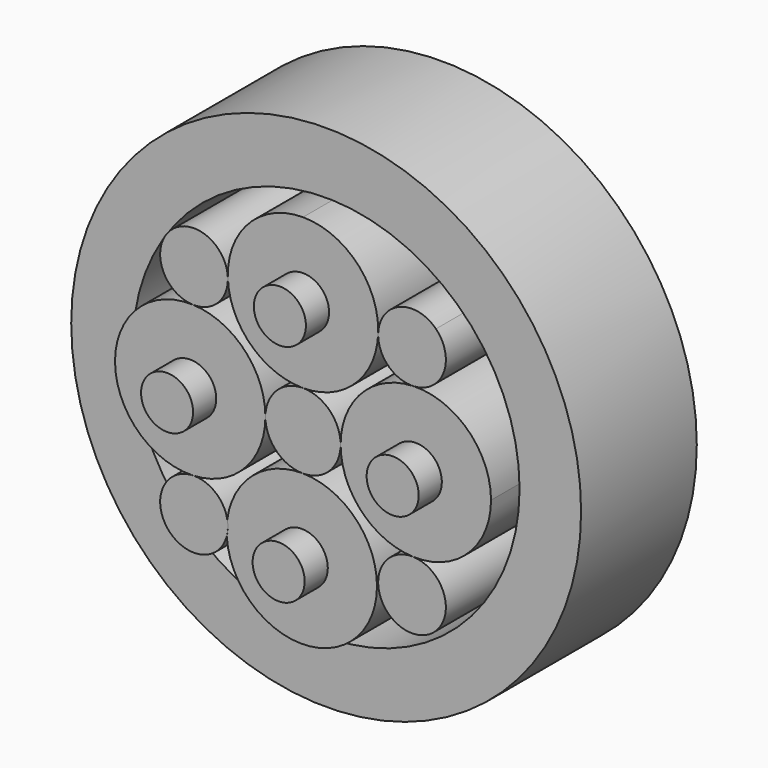
from build123d import *

# Parameters (mm, degrees)
F0_R      = 4.5
F1_DEPTH  = 35
F2_DEPTH  = 30
F3_DEPTH  = 30
F4_DEPTH  = 35
F5_DEPTH  = 30
F6_DEPTH  = 30
F7_DEPTH  = 35
F9_DEPTH  = 35
F10_R     = 44.074281088
F10_R_2   = 33.4370635173
F11_DEPTH = 25
F12_DEPTH = 30
F13_COUNT = 4
F14_DEPTH = 30


# Not quite as in the source:
# - a feature of the source that left no trace in its solid (it failed there, or was rolled back) is left out
# - a feature names something its author has since deleted; it is built from what else it names


with BuildPart() as f1:
    # F0 (on Front) → F1 (new body)
    with BuildSketch(Plane.XZ):
        with Locations((0, 19.5)):
            Circle(F0_R)
    extrude(amount=F1_DEPTH)


with BuildPart() as f2:
    # F0 (on Front) → F2 (new body)
    with BuildSketch(Plane.XZ):
        with BuildLine():
            ThreePointArc((-12.9920791749, 19.0462614041), (-9.030542571, 10.148566908), (0, 6.5))
            ThreePointArc((0, 6.5), (9.030542571, 10.148566908), (12.9920791749, 19.0462614041))
            ThreePointArc((12.9920791749, 19.0462614041), (12.9980196429, 19.2730961366), (13, 19.5))
            ThreePointArc((13, 19.5), (9.1923881501, 28.6923881607), (-1.5e-08, 32.5))
            ThreePointArc((-1.5e-08, 32.5), (-9.3514330972, 28.5305425656), (-12.9920791749, 19.0462614041))
        make_face()
        with Locations((0, 19.5)):
            Circle(F0_R, mode=Mode.SUBTRACT)
    extrude(amount=F2_DEPTH)


with BuildPart() as f3:
    # F0 (on Front) → F3 (new body)
    with BuildSketch(Plane.XZ):
        with BuildLine():
            ThreePointArc((-19.0462616463, -12.9920791833), (-10.1485669922, -9.0305426582), (-6.5, 0))
            ThreePointArc((-6.5, 0), (-10.1485669922, 9.0305426582), (-19.0462616463, 12.9920791833))
            ThreePointArc((-19.0462616463, 12.9920791833), (-28.5305425766, 9.3514330866), (-32.5, 2.269e-07))
            ThreePointArc((-32.5, 2.269e-07), (-28.5305427398, -9.351432929), (-19.0462616463, -12.9920791833))
        make_face()
        with Locations((-19.5, 0)):
            Circle(F0_R, mode=Mode.SUBTRACT)
    extrude(amount=F3_DEPTH)


with BuildPart() as f4:
    # F0 (on Front) → F4 (new body)
    with BuildSketch(Plane.XZ):
        with Locations((-19.5, 0)):
            Circle(F0_R)
    extrude(amount=F4_DEPTH)


with BuildPart() as f5:
    # F0 (on Front) → F5 (new body)
    with BuildSketch(Plane.XZ):
        with BuildLine():
            ThreePointArc((19.0462612866, 12.9920791708), (10.1485668672, 9.0305425287), (6.5, 0))
            ThreePointArc((6.5, 0), (10.1485669557, -9.0305426203), (19.0462615412, -12.9920791797))
            ThreePointArc((19.0462615412, -12.9920791797), (28.5305426203, -9.3514330443), (32.5, 0))
            ThreePointArc((32.5, 0), (28.5305425287, 9.3514331328), (19.0462612866, 12.9920791708))
        make_face()
        with Locations((19.5, 0)):
            Circle(F0_R, mode=Mode.SUBTRACT)
    extrude(amount=F5_DEPTH)


with BuildPart() as f6:
    # F0 (on Front) → F6 (new body)
    with BuildSketch(Plane.XZ):
        with BuildLine():
            ThreePointArc((12.7868825893, -19.4988353747), (9.0293664927, -10.3568174741), (-0.0710391484, -6.4996117914))
            ThreePointArc((-0.0710391484, -6.4996117914), (-8.706943876, -9.6573460577), (-13.0934155612, -17.7387445948))
            ThreePointArc((-13.0934155612, -17.7387445948), (-13.0147974373, -18.2878635968), (-12.9885127088, -18.8419588962))
            ThreePointArc((-12.9885127088, -18.8419588962), (-13.0379426477, -19.6010555008), (-13.1853976333, -20.34733159))
            ThreePointArc((-13.1853976333, -20.34733159), (-9.1521689219, -28.9377631782), (-0.355195428, -32.4980589606))
            ThreePointArc((-0.355195428, -32.4980589606), (8.928900577, -28.7413191919), (12.7868825893, -19.4988353747))
        make_face()
        with Locations((-0.2131174107, -19.4988353747)):
            Circle(F0_R, mode=Mode.SUBTRACT)
    extrude(amount=F6_DEPTH)


with BuildPart() as f7:
    # F0 (on Front) → F7 (new body)
    with BuildSketch(Plane.XZ):
        with Locations((19.5, 0)):
            Circle(F0_R)
    extrude(amount=F7_DEPTH)


with BuildPart() as f9:
    # F0 (on Front) → F9 (new body)
    with BuildSketch(Plane.XZ):
        with Locations((-0.2131174107, -19.4988353747)):
            Circle(F0_R)
    extrude(amount=F9_DEPTH)


with BuildPart() as f11:
    # F10 (on Front) → F11 (new body)
    with BuildSketch(Plane.XZ):
        Circle(F10_R)
        Circle(F10_R_2, mode=Mode.SUBTRACT)
    extrude(amount=F11_DEPTH)


with BuildPart() as f12:
    # F0 (on Front) → F12 (new body)
    with BuildSketch(Plane.XZ):
        with BuildLine():
            ThreePointArc((-12.9885127088, 18.8419588962), (-12.9894043933, 18.9441257137), (-12.9920791749, 19.0462614041))
            ThreePointArc((-12.9920791749, 19.0462614041), (-16.6966730995, 24.2881117694), (-22.9809704144, 22.9809703627))
            ThreePointArc((-22.9809704144, 22.9809703627), (-24.2881118005, 16.6966731783), (-19.0462616463, 12.9920791833))
            ThreePointArc((-19.0462616463, 12.9920791833), (-14.7758208566, 14.6313349862), (-12.9885127088, 18.8419588962))
        make_face()
    extrude(amount=F12_DEPTH)


with BuildPart() as f13_1:
    # F13: instance of F12
    add(f12.part.rotate(Axis((0, 0, 0), (0, -1, 0)), 1 * 360 / F13_COUNT))


with BuildPart() as f13_2:
    # F13: instance of F12
    add(f12.part.rotate(Axis((0, 0, 0), (0, -1, 0)), 2 * 360 / F13_COUNT))


with BuildPart() as f13_3:
    # F13: instance of F12
    add(f12.part.rotate(Axis((0, 0, 0), (0, -1, 0)), 3 * 360 / F13_COUNT))


with BuildPart() as f14:
    # F0 (on Front) → F14 (new body)
    with BuildSketch(Plane.XZ):
        with BuildLine():
            ThreePointArc((-0.0710391484, -6.4996117914), (4.5710089442, -4.6212419578), (6.5, 0))
            ThreePointArc((6.5, 0), (4.5961940777, 4.5961940777), (0, 6.5))
            ThreePointArc((0, 6.5), (-4.5961940777, 4.5961940777), (-6.5, 0))
            ThreePointArc((-6.5, 0), (-4.6212419578, -4.5710089442), (-0.0710391484, -6.4996117914))
        make_face()
    extrude(amount=F14_DEPTH)


solid = Compound([f1.part, f2.part, f3.part, f4.part, f5.part, f6.part, f7.part, f9.part, f11.part, f12.part, f13_1.part, f13_2.part, f13_3.part, f14.part])
